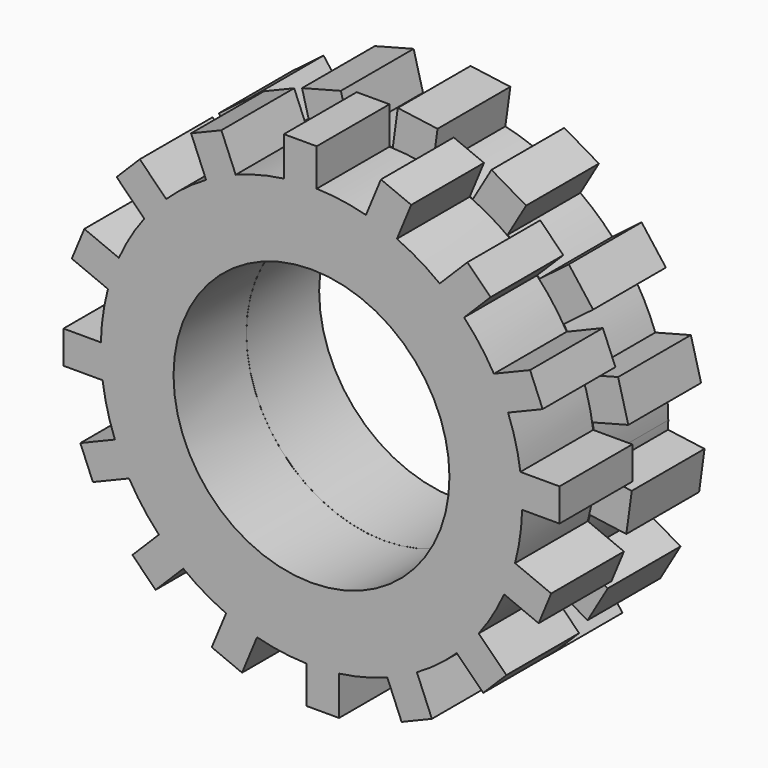
from build123d import *

# Parameters (mm, degrees)
F0_R     = 4.125
F1_DEPTH = 2.72
F2_R     = 4.1231298437
F3_DEPTH = 2.72


with BuildPart() as f1:
    # F0 (on Front) → F1 (new body)
    with BuildSketch(Plane.XZ):
        with BuildLine():
            ThreePointArc((6.2980790564, -0.1555641345), (6.2995197458, -0.0777879971), (6.3, 0))
            ThreePointArc((6.3, 0), (6.2864411705, 0.4131070197), (6.2458230445, 0.8244358655))
            Line((6.2458230445, 0.8244358655), (6.2458230445, -0.1555641345))
            Line((6.2458230445, -0.1555641345), (6.2980790564, -0.1555641345))
        make_face()
        with BuildLine():
            ThreePointArc((6.2458230445, 0.8244358655), (6.2864411705, 0.4131070197), (6.3, 0))
            ThreePointArc((6.3, 0), (6.2995197458, -0.0777879971), (6.2980790564, -0.1555641345))
            Line((6.2980790564, -0.1555641345), (7.4158230445, -0.1555641345))
            Line((7.4158230445, -0.1555641345), (7.4158230445, 0.8244358655))
            Line((7.4158230445, 0.8244358655), (6.2458230445, 0.8244358655))
        make_face()
        with BuildLine():
            Line((6.2458230445, -0.1555641345), (6.2458230445, 0.8244358655))
            ThreePointArc((6.2458230445, 0.8244358655), (6.1047376873, 1.5563347226), (5.8781981513, 2.2664479907))
            Line((5.8781981513, 2.2664479907), (5.8299198915, 2.2464504808))
            Line((5.8299198915, 2.2464504808), (5.4548901278, 3.1518524226))
            ThreePointArc((5.4548901278, 3.1518524226), (5.0444586871, 3.7740477678), (4.5634148636, 4.3434139548))
            Line((4.5634148636, 4.3434139548), (4.5264642833, 4.3064633745))
            Line((4.5264642833, 4.3064633745), (3.8334996377, 4.99942802))
            ThreePointArc((3.8334996377, 4.99942802), (3.21620658, 5.4171962522), (2.5538930305, 5.7591345174))
            Line((2.5538930305, 5.7591345174), (2.5338955205, 5.7108562576))
            Line((2.5338955205, 5.7108562576), (1.6284935786, 6.0858860213))
            ThreePointArc((1.6284935786, 6.0858860213), (0.898316176, 6.2356257142), (0.1555641345, 6.2980790564))
            Line((0.1555641345, 6.2980790564), (0.1555641345, 6.2458230445))
            Line((0.1555641345, 6.2458230445), (-0.8244358655, 6.2458230445))
            ThreePointArc((-0.8244358655, 6.2458230445), (-1.5563347226, 6.1047376873), (-2.2664479907, 5.8781981513))
            Line((-2.2664479907, 5.8781981513), (-2.2464504808, 5.8299198915))
            Line((-2.2464504808, 5.8299198915), (-3.1518524226, 5.4548901278))
            ThreePointArc((-3.1518524226, 5.4548901278), (-3.7740477678, 5.0444586871), (-4.3434139548, 4.5634148636))
            Line((-4.3434139548, 4.5634148636), (-4.3064633745, 4.5264642833))
            Line((-4.3064633745, 4.5264642833), (-4.99942802, 3.8334996377))
            ThreePointArc((-4.99942802, 3.8334996377), (-5.4171962522, 3.21620658), (-5.7591345174, 2.5538930305))
            Line((-5.7591345174, 2.5538930305), (-5.7108562576, 2.5338955205))
            Line((-5.7108562576, 2.5338955205), (-6.0858860213, 1.6284935786))
            ThreePointArc((-6.0858860213, 1.6284935786), (-6.2356257142, 0.898316176), (-6.2980790564, 0.1555641345))
            Line((-6.2980790564, 0.1555641345), (-6.2458230445, 0.1555641345))
            Line((-6.2458230445, 0.1555641345), (-6.2458230445, -0.8244358655))
            ThreePointArc((-6.2458230445, -0.8244358655), (-6.1047376873, -1.5563347226), (-5.8781981513, -2.2664479907))
            Line((-5.8781981513, -2.2664479907), (-5.8299198915, -2.2464504808))
            Line((-5.8299198915, -2.2464504808), (-5.4548901278, -3.1518524226))
            ThreePointArc((-5.4548901278, -3.1518524226), (-5.0444586871, -3.7740477678), (-4.5634148636, -4.3434139548))
            Line((-4.5634148636, -4.3434139548), (-4.5264642833, -4.3064633745))
            Line((-4.5264642833, -4.3064633745), (-3.8334996377, -4.99942802))
            ThreePointArc((-3.8334996377, -4.99942802), (-3.21620658, -5.4171962522), (-2.5538930305, -5.7591345174))
            Line((-2.5538930305, -5.7591345174), (-2.5338955205, -5.7108562576))
            Line((-2.5338955205, -5.7108562576), (-1.6284935786, -6.0858860213))
            ThreePointArc((-1.6284935786, -6.0858860213), (-0.898316176, -6.2356257142), (-0.1555641345, -6.2980790564))
            Line((-0.1555641345, -6.2980790564), (-0.1555641345, -6.2458230445))
            Line((-0.1555641345, -6.2458230445), (0.8054847051, -6.2458230445))
            Line((0.8054847051, -6.2458230445), (0.8244358655, -6.2458230445))
            ThreePointArc((0.8244358655, -6.2458230445), (1.5563347226, -6.1047376873), (2.2664479907, -5.8781981513))
            Line((2.2664479907, -5.8781981513), (2.2464504808, -5.8299198915))
            Line((2.2464504808, -5.8299198915), (3.1518524226, -5.4548901278))
            ThreePointArc((3.1518524226, -5.4548901278), (3.7740477678, -5.0444586871), (4.3434139548, -4.5634148636))
            Line((4.3434139548, -4.5634148636), (4.3064633745, -4.5264642833))
            Line((4.3064633745, -4.5264642833), (4.99942802, -3.8334996377))
            ThreePointArc((4.99942802, -3.8334996377), (5.4171962522, -3.21620658), (5.7591345174, -2.5538930305))
            Line((5.7591345174, -2.5538930305), (5.7108562576, -2.5338955205))
            Line((5.7108562576, -2.5338955205), (6.0858860213, -1.6284935786))
            ThreePointArc((6.0858860213, -1.6284935786), (6.2356257142, -0.898316176), (6.2980790564, -0.1555641345))
            Line((6.2980790564, -0.1555641345), (6.2458230445, -0.1555641345))
        make_face()
        Circle(F0_R, mode=Mode.SUBTRACT)
        with BuildLine():
            Line((5.8299198915, 2.2464504808), (5.8781981513, 2.2664479907))
            ThreePointArc((5.8781981513, 2.2664479907), (5.6838110223, 2.7174054285), (5.4548901278, 3.1518524226))
            Line((5.4548901278, 3.1518524226), (5.8299198915, 2.2464504808))
        make_face()
        with BuildLine():
            ThreePointArc((5.4548901278, 3.1518524226), (5.6838110223, 2.7174054285), (5.8781981513, 2.2664479907))
            Line((5.8781981513, 2.2664479907), (6.9108589445, 2.6941900966))
            Line((6.9108589445, 2.6941900966), (6.5358291808, 3.5995920385))
            Line((6.5358291808, 3.5995920385), (5.4548901278, 3.1518524226))
        make_face()
        with BuildLine():
            Line((7.1668250743, -2.0762331945), (6.0858860213, -1.6284935786))
            ThreePointArc((6.0858860213, -1.6284935786), (5.9405571226, -2.0975655111), (5.7591345174, -2.5538930305))
            Line((5.7591345174, -2.5538930305), (6.7917953106, -2.9816351364))
            Line((6.7917953106, -2.9816351364), (7.1668250743, -2.0762331945))
        make_face()
        with BuildLine():
            ThreePointArc((5.7591345174, -2.5538930305), (5.9405571226, -2.0975655111), (6.0858860213, -1.6284935786))
            Line((6.0858860213, -1.6284935786), (5.7108562576, -2.5338955205))
            Line((5.7108562576, -2.5338955205), (5.7591345174, -2.5538930305))
        make_face()
        with BuildLine():
            Line((4.5264642833, 4.3064633745), (4.5634148636, 4.3434139548))
            ThreePointArc((4.5634148636, 4.3434139548), (4.2112506336, 4.6856555679), (3.8334996377, 4.99942802))
            Line((3.8334996377, 4.99942802), (4.5264642833, 4.3064633745))
        make_face()
        with BuildLine():
            ThreePointArc((3.8334996377, 4.99942802), (4.2112506336, 4.6856555679), (4.5634148636, 4.3434139548))
            Line((4.5634148636, 4.3434139548), (5.3537792173, 5.1337783084))
            Line((5.3537792173, 5.1337783084), (4.6608145717, 5.826742954))
            Line((4.6608145717, 5.826742954), (3.8334996377, 4.99942802))
        make_face()
        with BuildLine():
            Line((5.826742954, -4.6608145717), (4.99942802, -3.8334996377))
            ThreePointArc((4.99942802, -3.8334996377), (4.6856555679, -4.2112506336), (4.3434139548, -4.5634148636))
            Line((4.3434139548, -4.5634148636), (5.1337783084, -5.3537792173))
            Line((5.1337783084, -5.3537792173), (5.826742954, -4.6608145717))
        make_face()
        with BuildLine():
            ThreePointArc((4.3434139548, -4.5634148636), (4.6856555679, -4.2112506336), (4.99942802, -3.8334996377))
            Line((4.99942802, -3.8334996377), (4.3064633745, -4.5264642833))
            Line((4.3064633745, -4.5264642833), (4.3434139548, -4.5634148636))
        make_face()
        with BuildLine():
            Line((2.5338955205, 5.7108562576), (2.5538930305, 5.7591345174))
            ThreePointArc((2.5538930305, 5.7591345174), (2.0975655111, 5.9405571226), (1.6284935786, 6.0858860213))
            Line((1.6284935786, 6.0858860213), (2.5338955205, 5.7108562576))
        make_face()
        with BuildLine():
            ThreePointArc((1.6284935786, 6.0858860213), (2.0975655111, 5.9405571226), (2.5538930305, 5.7591345174))
            Line((2.5538930305, 5.7591345174), (2.9816351364, 6.7917953106))
            Line((2.9816351364, 6.7917953106), (2.0762331945, 7.1668250743))
            Line((2.0762331945, 7.1668250743), (1.6284935786, 6.0858860213))
        make_face()
        with BuildLine():
            Line((3.5995920385, -6.5358291808), (3.1518524226, -5.4548901278))
            ThreePointArc((3.1518524226, -5.4548901278), (2.7174054285, -5.6838110223), (2.2664479907, -5.8781981513))
            Line((2.2664479907, -5.8781981513), (2.6941900966, -6.9108589445))
            Line((2.6941900966, -6.9108589445), (3.5995920385, -6.5358291808))
        make_face()
        with BuildLine():
            ThreePointArc((2.2664479907, -5.8781981513), (2.7174054285, -5.6838110223), (3.1518524226, -5.4548901278))
            Line((3.1518524226, -5.4548901278), (2.2464504808, -5.8299198915))
            Line((2.2464504808, -5.8299198915), (2.2664479907, -5.8781981513))
        make_face()
        with BuildLine():
            Line((0.1555641345, 6.2458230445), (0.1555641345, 6.2980790564))
            ThreePointArc((0.1555641345, 6.2980790564), (-0.335454946, 6.2910627067), (-0.8244358655, 6.2458230445))
            Line((-0.8244358655, 6.2458230445), (0.1555641345, 6.2458230445))
        make_face()
        with BuildLine():
            ThreePointArc((-0.8244358655, 6.2458230445), (-0.335454946, 6.2910627067), (0.1555641345, 6.2980790564))
            Line((0.1555641345, 6.2980790564), (0.1555641345, 7.4158230445))
            Line((0.1555641345, 7.4158230445), (-0.8244358655, 7.4158230445))
            Line((-0.8244358655, 7.4158230445), (-0.8244358655, 6.2458230445))
        make_face()
        with BuildLine():
            Line((0.8244358655, -7.4158230445), (0.8244358655, -6.2458230445))
            ThreePointArc((0.8244358655, -6.2458230445), (0.8141996188, -6.2471656758), (0.8039611857, -6.2484915309))
            ThreePointArc((0.8039611857, -6.2484915309), (0.3251452209, -6.2916039756), (-0.1555641345, -6.2980790564))
            Line((-0.1555641345, -6.2980790564), (-0.1555641345, -7.4158230445))
            Line((-0.1555641345, -7.4158230445), (0.8244358655, -7.4158230445))
        make_face()
        with BuildLine():
            ThreePointArc((0.8039611857, -6.2484915309), (0.8141996188, -6.2471656758), (0.8244358655, -6.2458230445))
            Line((0.8244358655, -6.2458230445), (0.8054847051, -6.2458230445))
            Line((0.8054847051, -6.2458230445), (0.8039611857, -6.2484915309))
        make_face()
        with BuildLine():
            ThreePointArc((-0.1555641345, -6.2980790564), (0.3251452209, -6.2916039756), (0.8039611857, -6.2484915309))
            Line((0.8039611857, -6.2484915309), (0.8054847051, -6.2458230445))
            Line((0.8054847051, -6.2458230445), (-0.1555641345, -6.2458230445))
            Line((-0.1555641345, -6.2458230445), (-0.1555641345, -6.2980790564))
        make_face()
        with BuildLine():
            Line((-2.2464504808, 5.8299198915), (-2.2664479907, 5.8781981513))
            ThreePointArc((-2.2664479907, 5.8781981513), (-2.7174054285, 5.6838110223), (-3.1518524226, 5.4548901278))
            Line((-3.1518524226, 5.4548901278), (-2.2464504808, 5.8299198915))
        make_face()
        with BuildLine():
            ThreePointArc((-3.1518524226, 5.4548901278), (-2.7174054285, 5.6838110223), (-2.2664479907, 5.8781981513))
            Line((-2.2664479907, 5.8781981513), (-2.6941900966, 6.9108589445))
            Line((-2.6941900966, 6.9108589445), (-3.5995920385, 6.5358291808))
            Line((-3.5995920385, 6.5358291808), (-3.1518524226, 5.4548901278))
        make_face()
        with BuildLine():
            Line((-2.0762331945, -7.1668250743), (-1.6284935786, -6.0858860213))
            ThreePointArc((-1.6284935786, -6.0858860213), (-2.0975655111, -5.9405571226), (-2.5538930305, -5.7591345174))
            Line((-2.5538930305, -5.7591345174), (-2.9816351364, -6.7917953106))
            Line((-2.9816351364, -6.7917953106), (-2.0762331945, -7.1668250743))
        make_face()
        with BuildLine():
            ThreePointArc((-2.5538930305, -5.7591345174), (-2.0975655111, -5.9405571226), (-1.6284935786, -6.0858860213))
            Line((-1.6284935786, -6.0858860213), (-2.5338955205, -5.7108562576))
            Line((-2.5338955205, -5.7108562576), (-2.5538930305, -5.7591345174))
        make_face()
        with BuildLine():
            Line((-4.3064633745, 4.5264642833), (-4.3434139548, 4.5634148636))
            ThreePointArc((-4.3434139548, 4.5634148636), (-4.6856555679, 4.2112506336), (-4.99942802, 3.8334996377))
            Line((-4.99942802, 3.8334996377), (-4.3064633745, 4.5264642833))
        make_face()
        with BuildLine():
            ThreePointArc((-4.99942802, 3.8334996377), (-4.6856555679, 4.2112506336), (-4.3434139548, 4.5634148636))
            Line((-4.3434139548, 4.5634148636), (-5.1337783084, 5.3537792173))
            Line((-5.1337783084, 5.3537792173), (-5.826742954, 4.6608145717))
            Line((-5.826742954, 4.6608145717), (-4.99942802, 3.8334996377))
        make_face()
        with BuildLine():
            Line((-4.6608145717, -5.826742954), (-3.8334996377, -4.99942802))
            ThreePointArc((-3.8334996377, -4.99942802), (-4.2112506336, -4.6856555679), (-4.5634148636, -4.3434139548))
            Line((-4.5634148636, -4.3434139548), (-5.3537792173, -5.1337783084))
            Line((-5.3537792173, -5.1337783084), (-4.6608145717, -5.826742954))
        make_face()
        with BuildLine():
            ThreePointArc((-4.5634148636, -4.3434139548), (-4.2112506336, -4.6856555679), (-3.8334996377, -4.99942802))
            Line((-3.8334996377, -4.99942802), (-4.5264642833, -4.3064633745))
            Line((-4.5264642833, -4.3064633745), (-4.5634148636, -4.3434139548))
        make_face()
        with BuildLine():
            Line((-5.7108562576, 2.5338955205), (-5.7591345174, 2.5538930305))
            ThreePointArc((-5.7591345174, 2.5538930305), (-5.9405571226, 2.0975655111), (-6.0858860213, 1.6284935786))
            Line((-6.0858860213, 1.6284935786), (-5.7108562576, 2.5338955205))
        make_face()
        with BuildLine():
            ThreePointArc((-6.0858860213, 1.6284935786), (-5.9405571226, 2.0975655111), (-5.7591345174, 2.5538930305))
            Line((-5.7591345174, 2.5538930305), (-6.7917953106, 2.9816351364))
            Line((-6.7917953106, 2.9816351364), (-7.1668250743, 2.0762331945))
            Line((-7.1668250743, 2.0762331945), (-6.0858860213, 1.6284935786))
        make_face()
        with BuildLine():
            Line((-6.5358291808, -3.5995920385), (-5.4548901278, -3.1518524226))
            ThreePointArc((-5.4548901278, -3.1518524226), (-5.6838110223, -2.7174054285), (-5.8781981513, -2.2664479907))
            Line((-5.8781981513, -2.2664479907), (-6.9108589445, -2.6941900966))
            Line((-6.9108589445, -2.6941900966), (-6.5358291808, -3.5995920385))
        make_face()
        with BuildLine():
            ThreePointArc((-5.8781981513, -2.2664479907), (-5.6838110223, -2.7174054285), (-5.4548901278, -3.1518524226))
            Line((-5.4548901278, -3.1518524226), (-5.8299198915, -2.2464504808))
            Line((-5.8299198915, -2.2464504808), (-5.8781981513, -2.2664479907))
        make_face()
        with BuildLine():
            Line((-6.2458230445, 0.1555641345), (-6.2980790564, 0.1555641345))
            ThreePointArc((-6.2980790564, 0.1555641345), (-6.2910627067, -0.335454946), (-6.2458230445, -0.8244358655))
            Line((-6.2458230445, -0.8244358655), (-6.2458230445, 0.1555641345))
        make_face()
        with BuildLine():
            ThreePointArc((-6.2458230445, -0.8244358655), (-6.2910627067, -0.335454946), (-6.2980790564, 0.1555641345))
            Line((-6.2980790564, 0.1555641345), (-7.4158230445, 0.1555641345))
            Line((-7.4158230445, 0.1555641345), (-7.4158230445, -0.8244358655))
            Line((-7.4158230445, -0.8244358655), (-6.2458230445, -0.8244358655))
        make_face()
    extrude(amount=F1_DEPTH)

    # F2 (on Front) → F3 (join)
    with BuildSketch(Plane.XZ):
        with BuildLine():
            ThreePointArc((6.310027427, -0.2555641345), (6.3139072063, -0.1278082441), (6.3152006426, 0))
            ThreePointArc((6.3152006426, 0), (6.2945166164, 0.5107051231), (6.2326000294, 1.0180648456))
            ThreePointArc((6.2326000294, 1.0180648456), (6.1076812308, 1.6056117651), (5.9275053496, 2.178632481))
            ThreePointArc((5.9275053496, 2.178632481), (5.6770845322, 2.7663098834), (5.3685750521, 3.3256820454))
            ThreePointArc((5.3685750521, 3.3256820454), (5.0283206589, 3.8207002641), (4.6425743157, 4.2811520506))
            ThreePointArc((4.6425743157, 4.2811520506), (4.1863212425, 4.7282632764), (3.6872331893, 5.1269943012))
            ThreePointArc((3.6872331893, 5.1269943012), (3.1834438485, 5.4541217827), (2.6508534272, 5.7319050292))
            ThreePointArc((2.6508534272, 5.7319050292), (2.0582284927, 5.9703814475), (1.4445434982, 6.147768151))
            ThreePointArc((1.4445434982, 6.147768151), (0.8539165702, 6.2572027015), (0.2555641345, 6.310027427))
            ThreePointArc((0.2555641345, 6.310027427), (-0.3832108872, 6.3035631648), (-1.0180648456, 6.2326000294))
            ThreePointArc((-1.0180648456, 6.2326000294), (-1.6056117651, 6.1076812308), (-2.178632481, 5.9275053496))
            ThreePointArc((-2.178632481, 5.9275053496), (-2.7663098834, 5.6770845322), (-3.3256820454, 5.3685750521))
            ThreePointArc((-3.3256820454, 5.3685750521), (-3.8207002641, 5.0283206589), (-4.2811520506, 4.6425743157))
            ThreePointArc((-4.2811520506, 4.6425743157), (-4.7282632764, 4.1863212425), (-5.1269943012, 3.6872331893))
            ThreePointArc((-5.1269943012, 3.6872331893), (-5.4541217827, 3.1834438485), (-5.7319050292, 2.6508534272))
            ThreePointArc((-5.7319050292, 2.6508534272), (-5.9703814475, 2.0582284927), (-6.147768151, 1.4445434982))
            ThreePointArc((-6.147768151, 1.4445434982), (-6.2572027015, 0.8539165702), (-6.310027427, 0.2555641345))
            ThreePointArc((-6.310027427, 0.2555641345), (-6.3035631648, -0.3832108872), (-6.2326000294, -1.0180648456))
            ThreePointArc((-6.2326000294, -1.0180648456), (-6.1076812308, -1.6056117651), (-5.9275053496, -2.178632481))
            ThreePointArc((-5.9275053496, -2.178632481), (-5.6770845322, -2.7663098834), (-5.3685750521, -3.3256820454))
            ThreePointArc((-5.3685750521, -3.3256820454), (-5.0283206589, -3.8207002641), (-4.6425743157, -4.2811520506))
            ThreePointArc((-4.6425743157, -4.2811520506), (-4.1863212425, -4.7282632764), (-3.6872331893, -5.1269943012))
            ThreePointArc((-3.6872331893, -5.1269943012), (-3.1834438485, -5.4541217827), (-2.6508534272, -5.7319050292))
            ThreePointArc((-2.6508534272, -5.7319050292), (-2.0582284927, -5.9703814475), (-1.4445434982, -6.147768151))
            ThreePointArc((-1.4445434982, -6.147768151), (-0.8539165702, -6.2572027015), (-0.2555641345, -6.310027427))
            ThreePointArc((-0.2555641345, -6.310027427), (0.3832108872, -6.3035631648), (1.0180648456, -6.2326000294))
            ThreePointArc((1.0180648456, -6.2326000294), (1.6056117651, -6.1076812308), (2.178632481, -5.9275053496))
            ThreePointArc((2.178632481, -5.9275053496), (2.7663098834, -5.6770845322), (3.3256820454, -5.3685750521))
            ThreePointArc((3.3256820454, -5.3685750521), (3.8207002641, -5.0283206589), (4.2811520506, -4.6425743157))
            ThreePointArc((4.2811520506, -4.6425743157), (4.7282632764, -4.1863212425), (5.1269943012, -3.6872331893))
            ThreePointArc((5.1269943012, -3.6872331893), (5.4541217827, -3.1834438485), (5.7319050292, -2.6508534272))
            ThreePointArc((5.7319050292, -2.6508534272), (5.9703814475, -2.0582284927), (6.147768151, -1.4445434982))
            ThreePointArc((6.147768151, -1.4445434982), (6.2572027015, -0.8539165702), (6.310027427, -0.2555641345))
        make_face()
        Circle(F2_R, mode=Mode.SUBTRACT)
        with BuildLine():
            ThreePointArc((5.9275053496, 2.178632481), (6.1076812308, 1.6056117651), (6.2326000294, 1.0180648456))
            Line((6.2326000294, 1.0180648456), (7.2964536952, 1.2977349688))
            Line((7.2964536952, 1.2977349688), (6.9913590154, 2.4583026042))
            Line((6.9913590154, 2.4583026042), (5.9275053496, 2.178632481))
        make_face()
        with BuildLine():
            Line((7.3999251771, -0.4043018042), (6.310027427, -0.2555641345))
            ThreePointArc((6.310027427, -0.2555641345), (6.2572027015, -0.8539165702), (6.147768151, -1.4445434982))
            Line((6.147768151, -1.4445434982), (7.2376659011, -1.5932811679))
            Line((7.2376659011, -1.5932811679), (7.3999251771, -0.4043018042))
        make_face()
        with BuildLine():
            ThreePointArc((4.6425743157, 4.2811520506), (5.0283206589, 3.8207002641), (5.3685750521, 3.3256820454))
            Line((5.3685750521, 3.3256820454), (6.2444225568, 3.9911827204))
            Line((6.2444225568, 3.9911827204), (5.5184218204, 4.9466527256))
            Line((5.5184218204, 4.9466527256), (4.6425743157, 4.2811520506))
        make_face()
        with BuildLine():
            Line((6.6819198111, -3.2053549279), (5.7319050292, -2.6508534272))
            ThreePointArc((5.7319050292, -2.6508534272), (5.4541217827, -3.1834438485), (5.1269943012, -3.6872331893))
            Line((5.1269943012, -3.6872331893), (6.0770090831, -4.2417346899))
            Line((6.0770090831, -4.2417346899), (6.6819198111, -3.2053549279))
        make_face()
        with BuildLine():
            ThreePointArc((2.6508534272, 5.7319050292), (3.1834438485, 5.4541217827), (3.6872331893, 5.1269943012))
            Line((3.6872331893, 5.1269943012), (4.2417346899, 6.0770090831))
            Line((4.2417346899, 6.0770090831), (3.2053549279, 6.6819198111))
            Line((3.2053549279, 6.6819198111), (2.6508534272, 5.7319050292))
        make_face()
        with BuildLine():
            Line((4.9466527256, -5.5184218204), (4.2811520506, -4.6425743157))
            ThreePointArc((4.2811520506, -4.6425743157), (3.8207002641, -5.0283206589), (3.3256820454, -5.3685750521))
            Line((3.3256820454, -5.3685750521), (3.9911827204, -6.2444225568))
            Line((3.9911827204, -6.2444225568), (4.9466527256, -5.5184218204))
        make_face()
        with BuildLine():
            ThreePointArc((0.2555641345, 6.310027427), (0.8539165702, 6.2572027015), (1.4445434982, 6.147768151))
            Line((1.4445434982, 6.147768151), (1.5932811679, 7.2376659011))
            Line((1.5932811679, 7.2376659011), (0.4043018042, 7.3999251771))
            Line((0.4043018042, 7.3999251771), (0.2555641345, 6.310027427))
        make_face()
        with BuildLine():
            Line((2.4583026042, -6.9913590154), (2.178632481, -5.9275053496))
            ThreePointArc((2.178632481, -5.9275053496), (1.6056117651, -6.1076812308), (1.0180648456, -6.2326000294))
            Line((1.0180648456, -6.2326000294), (1.2977349688, -7.2964536952))
            Line((1.2977349688, -7.2964536952), (2.4583026042, -6.9913590154))
        make_face()
        with BuildLine():
            ThreePointArc((-2.178632481, 5.9275053496), (-1.6056117651, 6.1076812308), (-1.0180648456, 6.2326000294))
            Line((-1.0180648456, 6.2326000294), (-1.2977349688, 7.2964536952))
            Line((-1.2977349688, 7.2964536952), (-2.4583026042, 6.9913590154))
            Line((-2.4583026042, 6.9913590154), (-2.178632481, 5.9275053496))
        make_face()
        with BuildLine():
            Line((-0.4043018042, -7.3999251771), (-0.2555641345, -6.310027427))
            ThreePointArc((-0.2555641345, -6.310027427), (-0.8539165702, -6.2572027015), (-1.4445434982, -6.147768151))
            Line((-1.4445434982, -6.147768151), (-1.5932811679, -7.2376659011))
            Line((-1.5932811679, -7.2376659011), (-0.4043018042, -7.3999251771))
        make_face()
        with BuildLine():
            ThreePointArc((-4.2811520506, 4.6425743157), (-3.8207002641, 5.0283206589), (-3.3256820454, 5.3685750521))
            Line((-3.3256820454, 5.3685750521), (-3.9911827204, 6.2444225568))
            Line((-3.9911827204, 6.2444225568), (-4.9466527256, 5.5184218204))
            Line((-4.9466527256, 5.5184218204), (-4.2811520506, 4.6425743157))
        make_face()
        with BuildLine():
            Line((-3.2053549279, -6.6819198111), (-2.6508534272, -5.7319050292))
            ThreePointArc((-2.6508534272, -5.7319050292), (-3.1834438485, -5.4541217827), (-3.6872331893, -5.1269943012))
            Line((-3.6872331893, -5.1269943012), (-4.2417346899, -6.0770090831))
            Line((-4.2417346899, -6.0770090831), (-3.2053549279, -6.6819198111))
        make_face()
        with BuildLine():
            ThreePointArc((-5.7319050292, 2.6508534272), (-5.4541217827, 3.1834438485), (-5.1269943012, 3.6872331893))
            Line((-5.1269943012, 3.6872331893), (-6.0770090831, 4.2417346899))
            Line((-6.0770090831, 4.2417346899), (-6.6819198111, 3.2053549279))
            Line((-6.6819198111, 3.2053549279), (-5.7319050292, 2.6508534272))
        make_face()
        with BuildLine():
            Line((-5.5184218204, -4.9466527256), (-4.6425743157, -4.2811520506))
            ThreePointArc((-4.6425743157, -4.2811520506), (-5.0283206589, -3.8207002641), (-5.3685750521, -3.3256820454))
            Line((-5.3685750521, -3.3256820454), (-6.2444225568, -3.9911827204))
            Line((-6.2444225568, -3.9911827204), (-5.5184218204, -4.9466527256))
        make_face()
        with BuildLine():
            ThreePointArc((-6.310027427, 0.2555641345), (-6.2572027015, 0.8539165702), (-6.147768151, 1.4445434982))
            Line((-6.147768151, 1.4445434982), (-7.2376659011, 1.5932811679))
            Line((-7.2376659011, 1.5932811679), (-7.3999251771, 0.4043018042))
            Line((-7.3999251771, 0.4043018042), (-6.310027427, 0.2555641345))
        make_face()
        with BuildLine():
            Line((-6.9913590154, -2.4583026042), (-5.9275053496, -2.178632481))
            ThreePointArc((-5.9275053496, -2.178632481), (-6.1076812308, -1.6056117651), (-6.2326000294, -1.0180648456))
            Line((-6.2326000294, -1.0180648456), (-7.2964536952, -1.2977349688))
            Line((-7.2964536952, -1.2977349688), (-6.9913590154, -2.4583026042))
        make_face()
    extrude(amount=-F3_DEPTH)


solid = f1.part
